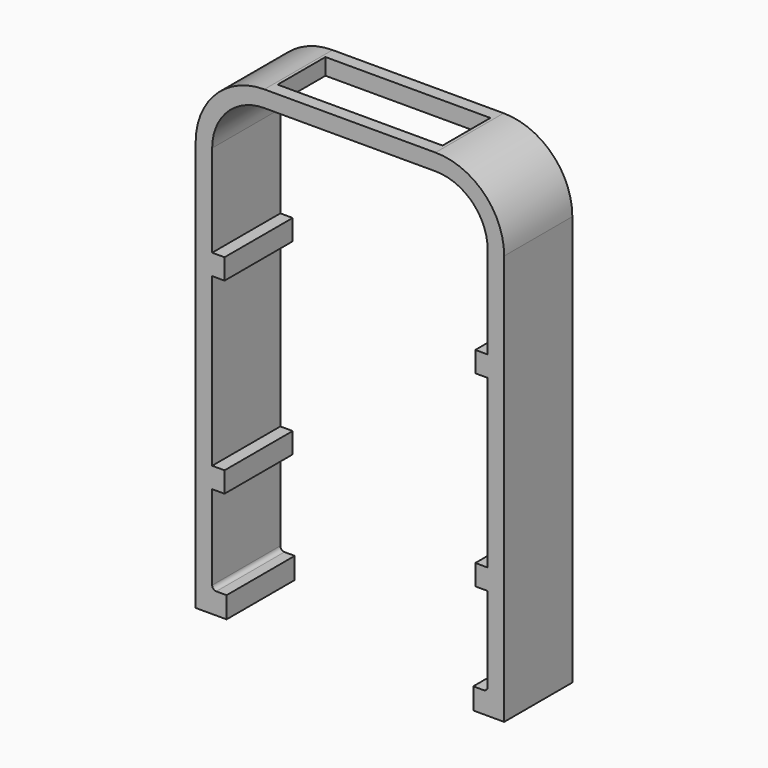
from build123d import *

# Parameters (mm, degrees)
F1_DEPTH     = 9.79181
F2_T         = -2.5
F3_R         = 5
F4_T1_DEPTH  = 80
F4_T3_DEPTH  = 40
F4_T6_ANGLE  = 90
F4_T8_ANGLE  = 90
F4_T10_ANGLE = 90
F4_T12_ANGLE = 90
F5_R         = 7
F6_R         = 4.5
F7_DEPTH     = 130
F8_T         = -2.5
F12_DEPTH    = 6.2
F13_R        = 0.3
F14_R        = 0.3
F15_W        = 12
F15_H        = 4.35
F16_DEPTH    = 67.90149


# Not quite as in the source:
# - a fillet or chamfer that OpenCascade refuses, or shapes differently, is made with other operations: its cross-section is extruded or revolved along the edge and cut away or added


with BuildPart() as f1:
    # F0 (on Front) → F1 (new body)
    with BuildSketch(Plane.XZ):
        with BuildLine():
            Line((33.4467580169, 25.7645070341), (-46.5532419831, 25.7645070341))
            ThreePointArc((-46.5532419831, 25.7645070341), (-50.088775889, 24.30004094), (-51.5532419831, 20.7645070341))
            Line((-51.5532419831, 20.7645070341), (-51.5532419831, -19.2354929659))
            ThreePointArc((-51.5532419831, -19.2354929659), (-50.088775889, -22.7710268718), (-46.5532419831, -24.2354929659))
            Line((-46.5532419831, -24.2354929659), (33.4467580169, -24.2354929659))
            ThreePointArc((33.4467580169, -24.2354929659), (36.9822919229, -22.7710268718), (38.4467580169, -19.2354929659))
            Line((38.4467580169, -19.2354929659), (38.4467580169, 20.7645070341))
            ThreePointArc((38.4467580169, 20.7645070341), (36.9822919229, 24.30004094), (33.4467580169, 25.7645070341))
        make_face()
    extrude(amount=F1_DEPTH)

    # F2
    f2_openings = [f1.faces().sort_by_distance(p)[0] for p in [
        (-6.553242, -9.79181, 0.764507),
    ]]
    offset(amount=F2_T, openings=f2_openings)

    # F3
    f3_edges = [f1.edges().sort_by_distance(p)[0] for p in [
        (-6.553242, -2.5, 23.264507),
    ]]
    fillet(f3_edges, radius=F3_R)

    # F4: fillet of radius 5 on 1 edges, made by hand

    # F4_s2 → F4_t1 (cut)
    with BuildSketch(Plane.YZ.offset(-46.5532419831)):
        with BuildLine():
            ThreePointArc((-6.145905, 23.0776584685), (-8.7774388713, 24.8717434082), (-9.79181, 27.890809903))
            Line((-9.79181, 27.890809903), (-10.29181, 27.890809903))
            Line((-10.29181, 27.890809903), (-10.29181, 23.2645070341))
            Line((-10.29181, 23.2645070341), (-9.79181, 22.7645070341))
            ThreePointArc((-9.79181, 22.7645070341), (-7.5, 22.7645070341), (-6.2813145, 22.5963433251))
            Line((-6.2813145, 22.5963433251), (-6.145905, 23.0776584685))
        make_face()
        with BuildLine():
            ThreePointArc((-9.79181, -26.3617958348), (-8.7774388713, -23.34272934), (-6.145905, -21.5486444004))
            Line((-6.145905, -21.5486444004), (-6.2813145, -21.0673292569))
            ThreePointArc((-6.2813145, -21.0673292569), (-7.5, -21.2354929659), (-9.79181, -21.2354929659))
            Line((-9.79181, -21.2354929659), (-10.29181, -21.7354929659))
            Line((-10.29181, -21.7354929659), (-10.29181, -26.3617958348))
            Line((-10.29181, -26.3617958348), (-9.79181, -26.3617958348))
        make_face()
    extrude(amount=F4_T1_DEPTH, mode=Mode.SUBTRACT)

    # F4_s4 → F4_t3 (cut)
    with BuildSketch(Plane.XY.offset(-19.2354929659)):
        with BuildLine():
            ThreePointArc((-53.679544852, -9.79181), (-50.6604783572, -8.7774388713), (-48.8663934175, -6.145905))
            Line((-48.8663934175, -6.145905), (-48.3850782741, -6.2813145))
            ThreePointArc((-48.3850782741, -6.2813145), (-48.5532419831, -7.5), (-48.5532419831, -9.79181))
            Line((-48.5532419831, -9.79181), (-49.0532419831, -10.29181))
            Line((-49.0532419831, -10.29181), (-53.679544852, -10.29181))
            Line((-53.679544852, -10.29181), (-53.679544852, -9.79181))
        make_face()
        with BuildLine():
            ThreePointArc((40.5730608858, -9.79181), (37.5539943911, -8.7774388713), (35.7599094514, -6.145905))
            Line((35.7599094514, -6.145905), (35.278594308, -6.2813145))
            ThreePointArc((35.278594308, -6.2813145), (35.4467580169, -7.5), (35.4467580169, -9.79181))
            Line((35.4467580169, -9.79181), (35.9467580169, -10.29181))
            Line((35.9467580169, -10.29181), (40.5730608858, -10.29181))
            Line((40.5730608858, -10.29181), (40.5730608858, -9.79181))
        make_face()
    extrude(amount=F4_T3_DEPTH, mode=Mode.SUBTRACT)

    # F4_s5 → F4_t6 (revolve, cut)
    with BuildSketch(Plane.XY.offset(20.7645070341)):
        with BuildLine():
            ThreePointArc((35.9467580169, -4.79181), (37.411224111, -8.3273439059), (40.9467580169, -9.79181))
            Line((40.9467580169, -9.79181), (40.9467580169, -9.89181))
            Line((40.9467580169, -9.89181), (35.8467580169, -9.89181))
            Line((35.8467580169, -9.89181), (35.8467580169, -4.79181))
            Line((35.8467580169, -4.79181), (35.9467580169, -4.79181))
        make_face()
    revolve(axis=Axis((33.4467580169, -9.79181, 20.7645070341), (0, -1, 0)), revolution_arc=F4_T6_ANGLE, mode=Mode.SUBTRACT)

    # F4_s7 → F4_t8 (revolve, cut)
    with BuildSketch(Plane.YZ.offset(-46.5532419831)):
        with BuildLine():
            ThreePointArc((-9.79181, 28.2645070341), (-8.3273439059, 24.7289731282), (-4.79181, 23.2645070341))
            Line((-4.79181, 23.2645070341), (-4.79181, 23.1645070341))
            Line((-4.79181, 23.1645070341), (-9.89181, 23.1645070341))
            Line((-9.89181, 23.1645070341), (-9.89181, 28.2645070341))
            Line((-9.89181, 28.2645070341), (-9.79181, 28.2645070341))
        make_face()
    revolve(axis=Axis((-46.5532419831, -9.79181, 20.7645070341), (0, -1, 0)), revolution_arc=F4_T8_ANGLE, mode=Mode.SUBTRACT)

    # F4_s9 → F4_t10 (revolve, cut)
    with BuildSketch(Plane.XY.offset(-19.2354929659)):
        with BuildLine():
            ThreePointArc((-54.0532419831, -9.79181), (-50.5177080771, -8.3273439059), (-49.0532419831, -4.79181))
            Line((-49.0532419831, -4.79181), (-48.9532419831, -4.79181))
            Line((-48.9532419831, -4.79181), (-48.9532419831, -9.89181))
            Line((-48.9532419831, -9.89181), (-54.0532419831, -9.89181))
            Line((-54.0532419831, -9.89181), (-54.0532419831, -9.79181))
        make_face()
    revolve(axis=Axis((-46.5532419831, -9.79181, -19.2354929659), (0, -1, 0)), revolution_arc=F4_T10_ANGLE, mode=Mode.SUBTRACT)

    # F4_s11 → F4_t12 (revolve, cut)
    with BuildSketch(Plane.YZ.offset(33.4467580169)):
        with BuildLine():
            ThreePointArc((-9.79181, -26.7354929659), (-8.3273439059, -23.19995906), (-4.79181, -21.7354929659))
            Line((-4.79181, -21.7354929659), (-4.79181, -21.6354929659))
            Line((-4.79181, -21.6354929659), (-9.89181, -21.6354929659))
            Line((-9.89181, -21.6354929659), (-9.89181, -26.7354929659))
            Line((-9.89181, -26.7354929659), (-9.79181, -26.7354929659))
        make_face()
    revolve(axis=Axis((33.4467580169, -9.79181, -19.2354929659), (0, -1, 0)), revolution_arc=F4_T12_ANGLE, mode=Mode.SUBTRACT)

    # F5
    f5_edges = [f1.edges().sort_by_distance(p)[0] for p in [
        (-6.553242, 0, 25.764507),
    ]]
    fillet(f5_edges, radius=F5_R)


with BuildPart() as f7:
    # F6 (on Front) → F7 (new body)
    with BuildSketch(Plane.XZ):
        with Locations((-6.3970589777, 0)):
            Circle(F6_R)
    extrude(amount=-F7_DEPTH)

    # F8
    f8_openings = [f7.faces().sort_by_distance(p)[0] for p in [
        (-6.397059, 130, 0),
    ]]
    offset(amount=F8_T, openings=f8_openings)


with BuildPart() as f12:
    # F11 (on Front) → F12 (new body)
    with BuildSketch(Plane.XZ):
        with BuildLine():
            Line((-43.4241547674, 46.4492497861), (-55.8741547674, 46.4492497861))
            ThreePointArc((-55.8741547674, 46.4492497861), (-59.4096886733, 44.9847836921), (-60.8741547674, 41.4492497861))
            Line((-60.8741547674, 41.4492497861), (-60.8741547674, 11.5992497861))
            Line((-60.8741547674, 11.5992497861), (-58.6241547674, 11.5992497861))
            Line((-58.6241547674, 11.5992497861), (-58.6241547674, 13.1492497861))
            Line((-58.6241547674, 13.1492497861), (-59.6741547674, 13.1492497861))
            Line((-59.6741547674, 13.1492497861), (-59.6741547674, 19.5992497861))
            Line((-59.6741547674, 19.5992497861), (-58.7741547674, 19.5992497861))
            Line((-58.7741547674, 19.5992497861), (-58.7741547674, 21.0992497861))
            Line((-58.7741547674, 21.0992497861), (-59.6741547674, 21.0992497861))
            Line((-59.6741547674, 21.0992497861), (-59.6741547674, 33.2492497861))
            Line((-59.6741547674, 33.2492497861), (-58.7741547674, 33.2492497861))
            Line((-58.7741547674, 33.2492497861), (-58.7741547674, 34.7492497861))
            Line((-58.7741547674, 34.7492497861), (-59.6741547674, 34.7492497861))
            Line((-59.6741547674, 34.7492497861), (-59.6741547674, 41.4492497861))
            ThreePointArc((-59.6741547674, 41.4492497861), (-58.5611605359, 44.1362555546), (-55.8741547674, 45.2492497861))
            Line((-55.8741547674, 45.2492497861), (-43.4241547674, 45.2492497861))
            ThreePointArc((-43.4241547674, 45.2492497861), (-40.7371489989, 44.1362555546), (-39.6241547674, 41.4492497861))
            Line((-39.6241547674, 41.4492497861), (-39.6241547674, 34.7492497861))
            Line((-39.6241547674, 34.7492497861), (-40.5241547674, 34.7492497861))
            Line((-40.5241547674, 34.7492497861), (-40.5241547674, 33.2492497861))
            Line((-40.5241547674, 33.2492497861), (-39.6241547674, 33.2492497861))
            Line((-39.6241547674, 33.2492497861), (-39.6241547674, 21.0992497861))
            Line((-39.6241547674, 21.0992497861), (-40.5241547674, 21.0992497861))
            Line((-40.5241547674, 21.0992497861), (-40.5241547674, 19.5992497861))
            Line((-40.5241547674, 19.5992497861), (-39.6241547674, 19.5992497861))
            Line((-39.6241547674, 19.5992497861), (-39.6241547674, 13.1492497861))
            Line((-39.6241547674, 13.1492497861), (-40.6741547674, 13.1492497861))
            Line((-40.6741547674, 13.1492497861), (-40.6741547674, 11.5992497861))
            Line((-40.6741547674, 11.5992497861), (-38.4241547674, 11.5992497861))
            Line((-38.4241547674, 11.5992497861), (-38.4241547674, 41.4492497861))
            ThreePointArc((-38.4241547674, 41.4492497861), (-39.8886208615, 44.9847836921), (-43.4241547674, 46.4492497861))
        make_face()
    extrude(amount=F12_DEPTH)

    # F13
    f13_edges = [f12.edges().sort_by_distance(p)[0] for p in [
        (-59.674155, -3.1, 13.14925),
    ]]
    fillet(f13_edges, radius=F13_R)

    # F14
    f14_edges = [f12.edges().sort_by_distance(p)[0] for p in [
        (-39.624155, -3.1, 13.14925),
    ]]
    fillet(f14_edges, radius=F14_R)

    # F15 (on Top) → F16 (cut)
    with BuildSketch(Plane.XY):
        with Locations((-49.6491547674, -3.1)):
            Rectangle(F15_W, F15_H)
    extrude(amount=F16_DEPTH, mode=Mode.SUBTRACT)


solid = f12.part
